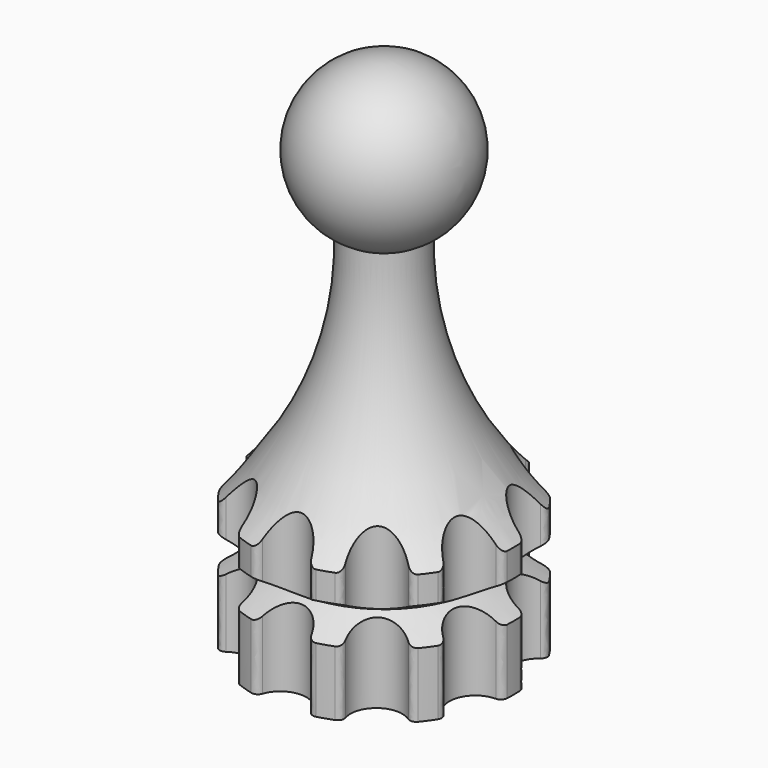
from build123d import *

# Parameters (mm, degrees)
F2_R            = 4
F3_DEPTH        = 25
F3_COPIES_COUNT = 10
F4_R            = 1


# Not quite as in the source:
# - a pattern or mirror of a feature is missing from the dataset's text; its kind, count and spacing are read off the source's solid


with BuildPart() as f1:
    # F0 (on Front) → F1 (revolve)
    with BuildSketch(Plane.XZ):
        with BuildLine():
            Line((0, 80), (0, 0))
            Line((0, 0), (20, 0))
            Line((20, 0), (20, 10))
            Line((20, 10), (15, 12.8867513459))
            Line((15, 12.8867513459), (20, 15.7735026919))
            Line((20, 15.7735026919), (20, 20))
            ThreePointArc((20, 20), (9.2929095445, 36.8536001431), (6.0343972867, 56.5530346951))
            ThreePointArc((6.0343972867, 56.5530346951), (12.1055166414, 70.6155203168), (0, 80))
        make_face()
    revolve(axis=Axis((0, 0, 25.6876507401), (0, 0, -1)))

    # F2 (on face) → F3 (cut)
    with BuildSketch(Plane(origin=(0, 0, 0), x_dir=(1, 0, 0), z_dir=(0, 0, -1))):
        with Locations((0.0077938561, 19.9999984814)):
            Circle(F2_R)
    f3 = extrude(amount=-F3_DEPTH, mode=Mode.SUBTRACT)

    # F3_copies: F3 ×10 about axis
    f3_copies_axis = Axis((0, 0, 0), (0, 0, 1))
    for i in range(1, F3_COPIES_COUNT):
        add(f3.rotate(f3_copies_axis, i * 360 / F3_COPIES_COUNT), mode=Mode.SUBTRACT)

    # F4
    f4_edges = [f1.edges().sort_by_distance(p)[0] for p in [
        (3.987587, -19.598448, 17.886751),
        (-3.972311, -19.601549, 17.886751),
        (3.987587, -19.598448, 5),
        (-3.972311, -19.601549, 5),
        (19.869693, 2.279319, 17.886751),
        (19.871464, -2.263832, 17.886751),
        (17.406999, 9.848674, 17.886751),
        (14.735169, 13.523121, 17.886751),
        (8.293652, 18.199322, 17.886751),
        (3.972311, 19.601549, 17.886751),
        (-3.987587, 19.598448, 17.886751),
        (-8.307834, 18.192853, 17.886751),
        (-14.745704, 13.511632, 17.886751),
        (-17.41467, 9.835105, 17.886751),
        (-19.871464, 2.263832, 17.886751),
        (-19.869693, -2.279319, 17.886751),
        (-17.406999, -9.848674, 17.886751),
        (-14.735169, -13.523121, 17.886751),
        (-8.293652, -18.199322, 17.886751),
        (8.307834, -18.192853, 17.886751),
        (14.745704, -13.511632, 17.886751),
        (17.41467, -9.835105, 17.886751),
        (8.307834, -18.192853, 5),
        (14.745704, -13.511632, 5),
        (17.41467, -9.835105, 5),
        (19.871464, -2.263832, 5),
        (19.869693, 2.279319, 5),
        (17.406999, 9.848674, 5),
        (14.735169, 13.523121, 5),
        (8.293652, 18.199322, 5),
        (3.972311, 19.601549, 5),
        (-3.987587, 19.598448, 5),
        (-8.307834, 18.192853, 5),
        (-14.745704, 13.511632, 5),
        (-17.41467, 9.835105, 5),
        (-19.871464, 2.263832, 5),
        (-19.869693, -2.279319, 5),
        (-17.406999, -9.848674, 5),
        (-14.735169, -13.523121, 5),
        (-8.293652, -18.199322, 5),
    ]]
    fillet(f4_edges, radius=F4_R)


solid = f1.part
